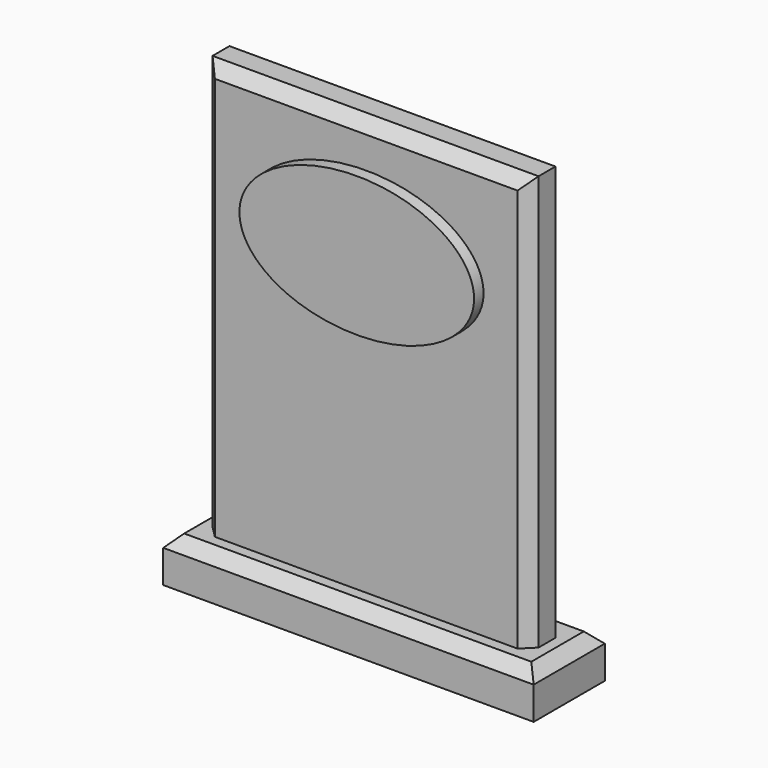
from build123d import *

# Parameters (mm, degrees)
F0_W     = 158.75
F0_H     = 38.1
F1_DEPTH = 19.05
F2_W     = 139.7
F2_H     = 19.05
F3_DEPTH = 177.8
F4_SIZE  = 5
F6_DEPTH = 5.08


with BuildPart() as f1:
    # F0 (on Top) → F1 (new body)
    with BuildSketch(Plane.XY):
        Rectangle(F0_W, F0_H)
    extrude(amount=F1_DEPTH)

    # F2 (on face) → F3 (join)
    with BuildSketch(Plane.XY.offset(19.05)):
        Rectangle(F2_W, F2_H)
    extrude(amount=F3_DEPTH)

    # F4
    f4_edges = [f1.edges().sort_by_distance(p)[0] for p in [
        (0, -19.05, 19.05),
        (-79.375, 0, 19.05),
        (79.375, 0, 19.05),
        (0, 19.05, 19.05),
        (-69.85, -9.525, 107.95),
        (-69.85, 9.525, 107.95),
        (0, -9.525, 196.85),
        (0, 9.525, 196.85),
        (69.85, -9.525, 107.95),
        (69.85, 9.525, 107.95),
    ]]
    chamfer(f4_edges, length=F4_SIZE)


with BuildPart() as f6:
    # F5 (on face) → F6 (new body)
    with BuildSketch(Plane.XZ.offset(9.525)):
        with BuildLine():
            add(Edge.make_bspline(
                [(50.2747856081, 148.3674943447), (50.2747856081, 200.3290185718), (-25.137392804, 174.3482564582), (-100.5495712161, 148.3674943447), (-25.137392804, 122.3867322312), (50.2747856081, 96.4059701176), (50.2747856081, 148.3674943447)],
                knots=[0, 0, 0, 2.0943951024, 2.0943951024, 4.1887902048, 4.1887902048, 6.2831853072, 6.2831853072, 6.2831853072], degree=2, weights=[1, 0.5, 1, 0.5, 1, 0.5, 1]))
        make_face()
    extrude(amount=F6_DEPTH)


solid = Compound([f1.part, f6.part])
